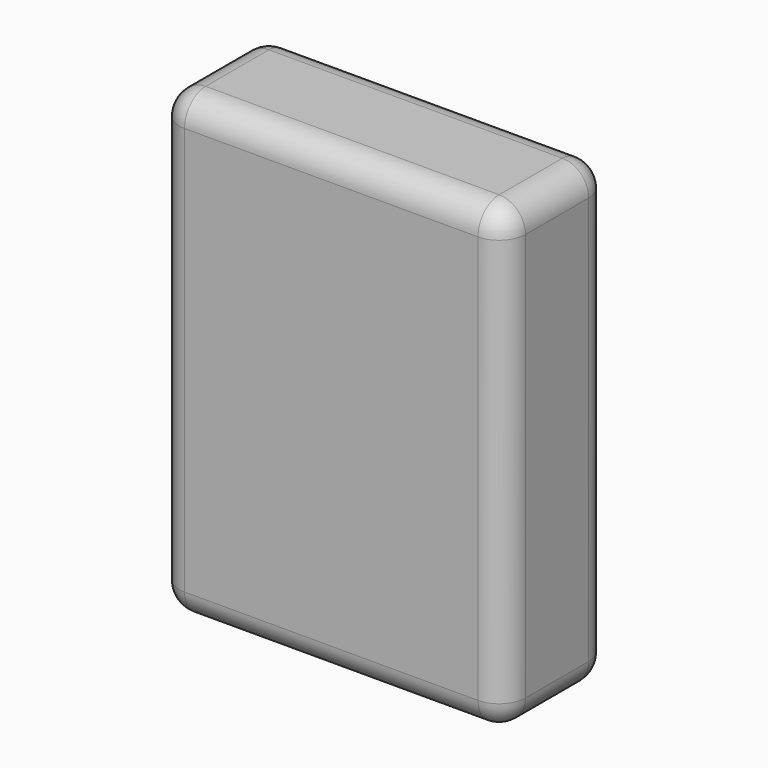
from build123d import *

# Parameters (mm, degrees)
F0_W     = 66.714566201
F0_H     = 88.7944847345
F1_DEPTH = 25.4
F2_R     = 5.08
F3_R     = 2.1888893323
F4_DEPTH = 1.27
F5_R     = 0.63499


# Not quite as in the source:
# - a fillet or chamfer is up to 0.001 mm smaller than in the source, because OpenCascade refuses the exact size


with BuildPart() as f1:
    # F0 (on Front) → F1 (new body)
    with BuildSketch(Plane.XZ):
        with Locations((0.118708238, -3.5612769425)):
            Rectangle(F0_W, F0_H)
    extrude(amount=F1_DEPTH)

    # F2
    f2_edges = [f1.edges().sort_by_distance(p)[0] for p in [
        (33.475991, -25.4, -3.561277),
        (0.118708, -25.4, -47.958519),
        (33.475991, -12.7, -47.958519),
        (33.475991, -12.7, 40.835965),
        (33.475991, 0, -3.561277),
        (0.118708, -25.4, 40.835965),
        (-33.238575, -12.7, 40.835965),
        (-33.238575, -12.7, -47.958519),
        (-33.238575, 0, -3.561277),
        (-33.238575, -25.4, -3.561277),
        (0.118708, 0, 40.835965),
        (0.118708, 0, -47.958519),
    ]]
    fillet(f2_edges, radius=F2_R)

    # F3 (on face) → F4 (join)
    with BuildSketch(Plane(origin=(0, 0, -47.9585193098), x_dir=(1, 0, 0), z_dir=(0, 0, -1))):
        with Locations((-20.655401051, 16.3818709552)):
            Circle(F3_R)
    extrude(amount=F4_DEPTH)

    # F5 (radius 0.635 in the source; OpenCascade refuses exactly that, so slightly less here)
    f5_edges = [f1.edges().sort_by_distance(p)[0] for p in [
        (-22.84429, -16.381871, -49.228519),
        (-22.84429, -16.381871, -47.958519),
        (-18.466512, -16.381871, -48.593519),
    ]]
    fillet(f5_edges, radius=F5_R)


solid = f1.part
